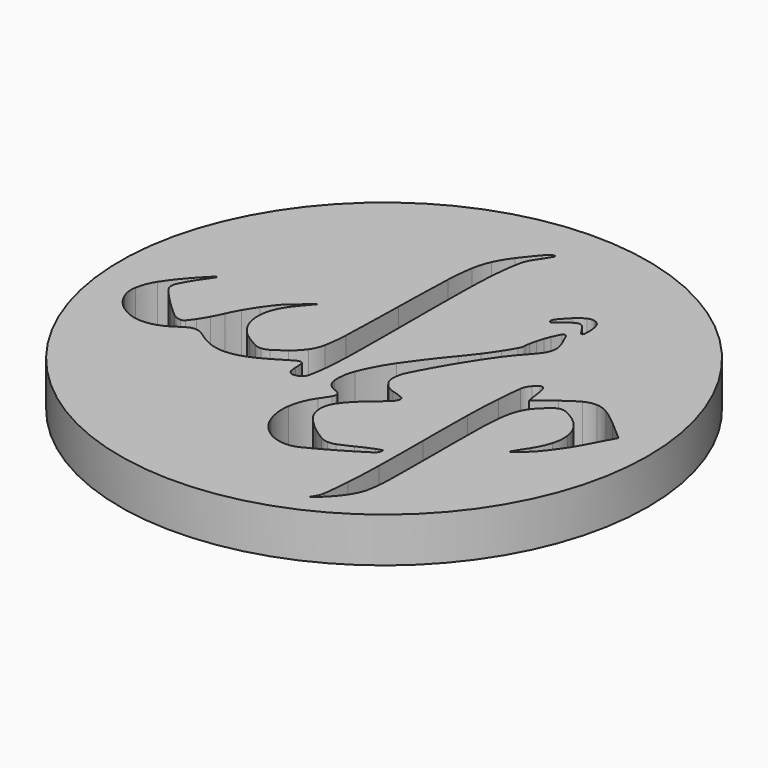
from build123d import *

# Parameters (mm, degrees)
F0_R     = 37.4493495169
F1_DEPTH = 6.35


# Not quite as in the source:
# - ends of sketch curves that miss each other by under 0.0002 mm in the source are joined


with BuildPart() as f1:
    # F0 (on Top) → F1 (new body)
    with BuildSketch(Plane.XY):
        Circle(F0_R)
        with BuildLine():
            ThreePointArc((10.8762792992, 14.7634018997), (11.0313140513, 15.1945068604), (11.2048912988, 15.61848587))
            ThreePointArc((11.2048912988, 15.61848587), (11.4768149901, 16.2225478114), (11.7640170164, 16.8194969919))
            ThreePointArc((11.7640170164, 16.8194969919), (11.8893481048, 16.9475361559), (12.0659669633, 16.9776647483))
            ThreePointArc((12.0659669633, 16.9776647483), (12.2485562258, 16.9031054882), (12.3751538129, 16.7518739087))
            ThreePointArc((12.3751538129, 16.7518739087), (12.70768613, 16.0552130167), (13.0282612117, 15.3529696483))
            ThreePointArc((13.0282612117, 15.3529696483), (13.2526035183, 14.7629142618), (13.4091322236, 14.151364044))
            ThreePointArc((13.4091322236, 14.151364044), (13.4527191197, 13.6473123792), (13.3873230886, 13.1456239785))
            ThreePointArc((13.3873230886, 13.1456239785), (13.20788262, 12.622156364), (12.9350425168, 12.1407256401))
            ThreePointArc((12.9350425168, 12.1407256401), (12.4654497003, 11.5128213922), (11.954437155, 10.9181388574))
            ThreePointArc((11.954437155, 10.9181388574), (10.5977208323, 9.3370006294), (9.3535167188, 7.6658831946))
            ThreePointArc((9.3535167188, 7.6658831946), (7.9199939418, 5.5117752747), (6.5659491385, 3.3068419184))
            ThreePointArc((6.5659491385, 3.3068419184), (5.3561218351, 1.1848137262), (4.2075785231, -0.9710002691))
            ThreePointArc((4.2075785231, -0.9710002691), (3.8216929788, -2.0075200449), (3.690609, -3.105745))
            ThreePointArc((3.690609, -3.105745), (3.7283068737, -3.4979838686), (3.8400200101, -3.8758629959))
            ThreePointArc((3.8400200101, -3.8758629959), (4.0285012326, -4.2562241711), (4.272961992, -4.6032670066))
            ThreePointArc((4.272961992, -4.6032670066), (4.574824271, -4.917630684), (4.9200760102, -5.1836129845))
            ThreePointArc((4.9200760102, -5.1836129845), (5.2913337091, -5.3865761409), (5.6906089952, -5.5265960184))
            ThreePointArc((5.6906089952, -5.5265960184), (6.4648720842, -5.7622274602), (7.2180381288, -6.0584477071))
            ThreePointArc((7.2180381288, -6.0584477071), (7.4657520558, -6.2976772359), (7.498624445, -6.6404778535))
            ThreePointArc((7.498624445, -6.6404778535), (7.3057418512, -7.0923112563), (6.9913608485, -7.4698318311))
            ThreePointArc((6.9913608485, -7.4698318311), (5.822940269, -8.5010016157), (4.6384584815, -9.5136815722))
            ThreePointArc((4.6384584815, -9.5136815722), (3.5443912184, -10.5668326908), (2.6004474224, -11.7564042914))
            ThreePointArc((2.6004474224, -11.7564042914), (2.1120521618, -12.7752539981), (1.962080368, -13.8951169912))
            ThreePointArc((1.962080368, -13.8951169912), (2.1657330329, -15.0003544038), (2.7035807171, -15.9871392184))
            ThreePointArc((2.7035807171, -15.9871392184), (3.7010773675, -17.1109770699), (4.8426470957, -18.0881308713))
            ThreePointArc((4.8426470957, -18.0881308713), (5.6504419064, -18.6581957262), (6.4856560106, -19.1872739822))
            ThreePointArc((6.4856560106, -19.1872739822), (7.0039493082, -19.4207975991), (7.5621359772, -19.5284493064))
            ThreePointArc((7.5621359772, -19.5284493064), (8.1400728978, -19.506565557), (8.6987199814, -19.3568879527))
            ThreePointArc((8.6987199814, -19.3568879527), (9.6550491416, -18.9570661492), (10.5926469221, -18.5151008439))
            ThreePointArc((10.5926469221, -18.5151008439), (11.1841988634, -18.2269156279), (11.7810690718, -17.9499131586))
            ThreePointArc((11.7810690718, -17.9499131586), (12.2773531843, -17.7352351951), (12.7805830392, -17.5373861048))
            ThreePointArc((12.7805830392, -17.5373861048), (13.1715302022, -17.3967091194), (13.5658320421, -17.2657291322))
            ThreePointArc((13.5658320421, -17.2657291322), (13.6513741496, -17.2796593868), (13.690609, -17.356939))
            ThreePointArc((13.690609, -17.356939), (13.5507780415, -17.9021018073), (13.1658118907, -18.3126578281))
            ThreePointArc((13.1658118907, -18.3126578281), (11.4102059781, -19.4044531735), (9.6328741998, -20.4605123442))
            ThreePointArc((9.6328741998, -20.4605123442), (7.8688014367, -21.4508314838), (6.0767982834, -22.3896655605))
            ThreePointArc((6.0767982834, -22.3896655605), (5.2070875666, -22.7082001651), (4.287215, -22.816345))
            ThreePointArc((4.287215, -22.816345), (2.6899630934, -22.5565730644), (1.2573490722, -21.804035904))
            ThreePointArc((1.2573490722, -21.804035904), (0.0637639813, -20.6069080986), (-0.7466320594, -19.1233250222))
            ThreePointArc((-0.7466320594, -19.1233250222), (-1.1677453841, -17.3401224067), (-1.1306904032, -15.5082449406))
            ThreePointArc((-1.1306904032, -15.5082449406), (-0.6419235107, -13.6890343723), (0.2526270965, -12.0312650676))
            ThreePointArc((0.2526270965, -12.0312650676), (0.7024614657, -11.3697564368), (1.1338345481, -10.6960637194))
            ThreePointArc((1.1338345481, -10.6960637194), (1.2685581494, -10.3917546236), (1.314644, -10.062163))
            ThreePointArc((1.314644, -10.062163), (1.2505882613, -9.810269569), (1.0739838069, -9.6195752982))
            ThreePointArc((1.0739838069, -9.6195752982), (0.6741945934, -9.38926579), (0.252626854, -9.2017703805))
            ThreePointArc((0.252626854, -9.2017703805), (-0.6381425922, -8.5264459955), (-1.0293586268, -7.4793150473))
            ThreePointArc((-1.0293586268, -7.4793150473), (-0.9713565511, -5.919909632), (-0.5670643499, -4.4127078625))
            ThreePointArc((-0.5670643499, -4.4127078625), (0.4843111612, -2.1378621147), (1.7936783431, -0.0010722388))
            ThreePointArc((1.7936783431, -0.0010722388), (3.8757468093, 2.856172185), (6.0790169795, 5.621033017))
            ThreePointArc((6.0790169795, 5.621033017), (6.8827913662, 6.6129347591), (7.6597352065, 7.625989846))
            ThreePointArc((7.6597352065, 7.625989846), (8.3503282831, 8.5851668879), (9.0081988691, 9.5670760845))
            ThreePointArc((9.0081988691, 9.5670760845), (9.526996254, 10.3975433886), (10.0205543041, 11.2432543922))
            ThreePointArc((10.0205543041, 11.2432543922), (10.199239966, 11.6673986677), (10.27697651, 12.1210329718))
            ThreePointArc((10.27697651, 12.1210329718), (10.3103188192, 12.490680364), (10.3692449003, 12.857120823))
            ThreePointArc((10.3692449003, 12.857120823), (10.4695885331, 13.3268146141), (10.585177224, 13.7929909406))
            ThreePointArc((10.585177224, 13.7929909406), (10.7229395483, 14.2805328648), (10.8762792992, 14.7634018997))
        make_face(mode=Mode.SUBTRACT)
        with BuildLine():
            ThreePointArc((16.3309902954, 3.7992979617), (16.5333642735, 4.4728969515), (16.9406093287, 5.0463446746))
            ThreePointArc((16.9406093287, 5.0463446746), (17.2598056295, 5.343826229), (17.6018882418, 5.6146786679))
            ThreePointArc((17.6018882418, 5.6146786679), (17.7996980335, 5.687411325), (18.0061756932, 5.6451534092))
            ThreePointArc((18.0061756932, 5.6451534092), (18.1901775594, 5.4936170925), (18.2964146053, 5.2802308984))
            ThreePointArc((18.2964146053, 5.2802308984), (18.4172751076, 4.757844237), (18.512282531, 4.2301429274))
            Line((18.512282531, 4.2301429274), (18.833957, 2.151252))
            Line((18.833957, 2.151252), (21.397142, 4.167454))
            ThreePointArc((21.397142, 4.167454), (22.4923393479, 4.9580300918), (23.6489884371, 5.6556192026))
            ThreePointArc((23.6489884371, 5.6556192026), (24.4741003602, 5.9692708509), (25.3534839934, 6.0458978723))
            ThreePointArc((25.3534839934, 6.0458978723), (26.2473925362, 5.8817071), (27.0687353681, 5.4925705707))
            ThreePointArc((27.0687353681, 5.4925705707), (28.2571790367, 4.6657006768), (29.3848450562, 3.757691065))
            Line((29.3848450562, 3.757691065), (32.190609, 1.331727))
            Line((32.190609, 1.331727), (30.296248, -2.217966))
            ThreePointArc((30.296248, -2.217966), (29.8748039715, -2.9711936195), (29.4237215636, -3.7070547204))
            ThreePointArc((29.4237215636, -3.7070547204), (28.9078737011, -4.4849173273), (28.3677878465, -5.2461508874))
            ThreePointArc((28.3677878465, -5.2461508874), (27.8427259014, -5.9385103963), (27.2957506754, -6.6136917283))
            ThreePointArc((27.2957506754, -6.6136917283), (26.8611052315, -7.0949015101), (26.3914461694, -7.5420031919))
            ThreePointArc((26.3914461694, -7.5420031919), (25.6864160048, -8.1620933021), (24.979266979, -8.7797659759))
            ThreePointArc((24.979266979, -8.7797659759), (24.9099925614, -8.7951216813), (24.8594533271, -8.7453169008))
            ThreePointArc((24.8594533271, -8.7453169008), (24.8509309758, -8.637712529), (24.8881566091, -8.5363933884))
            ThreePointArc((24.8881566091, -8.5363933884), (25.4995896841, -7.5796648027), (26.1129343447, -6.6241605785))
            ThreePointArc((26.1129343447, -6.6241605785), (26.7661686916, -5.4325781155), (27.2462296984, -4.1613089097))
            ThreePointArc((27.2462296984, -4.1613089097), (27.4657691357, -2.9950770933), (27.4378427219, -1.8086899068))
            ThreePointArc((27.4378427219, -1.8086899068), (27.1700390601, -0.7322913639), (26.6628924871, 0.2541946563))
            ThreePointArc((26.6628924871, 0.2541946563), (25.9198905189, 1.1553031996), (25.0139108115, 1.8923577146))
            ThreePointArc((25.0139108115, 1.8923577146), (24.3770565009, 2.28252617), (23.7150840631, 2.6283691314))
            ThreePointArc((23.7150840631, 2.6283691314), (23.2943006235, 2.7577930414), (22.8540629043, 2.7580246401))
            ThreePointArc((22.8540629043, 2.7580246401), (22.4102098559, 2.6293294742), (22.0161851262, 2.3878498451))
            ThreePointArc((22.0161851262, 2.3878498451), (21.3756572026, 1.8383388903), (20.7639108044, 1.2569571956))
            ThreePointArc((20.7639108044, 1.2569571956), (20.1177126912, 0.4779983542), (19.6265125546, -0.4069148044))
            ThreePointArc((19.6265125546, -0.4069148044), (19.2490785938, -1.4585132195), (19.0204482398, -2.552151033))
            ThreePointArc((19.0204482398, -2.552151033), (18.8311079762, -4.3239318853), (18.7496716179, -6.1039389941))
            ThreePointArc((18.7496716179, -6.1039389941), (18.7053745197, -9.9521401876), (18.690609, -13.800568))
            ThreePointArc((18.690609, -13.800568), (18.6766098173, -18.0136665407), (18.634611, -22.226579))
            ThreePointArc((18.634611, -22.226579), (18.5483521208, -23.8515074769), (18.3333395333, -25.4644559188))
            ThreePointArc((18.3333395333, -25.4644559188), (18.0420774391, -26.532147306), (17.5563022349, -27.5265421435))
            ThreePointArc((17.5563022349, -27.5265421435), (16.8067801698, -28.6115975468), (15.9406085284, -29.6060195403))
            ThreePointArc((15.9406085284, -29.6060195403), (15.4455501352, -30.1087206825), (14.9453633663, -30.606319372))
            ThreePointArc((14.9453633663, -30.606319372), (14.6624168408, -30.8702392299), (14.3656094129, -31.1184685217))
            ThreePointArc((14.3656094129, -31.1184685217), (14.3129853823, -31.1201666484), (14.2959902827, -31.0703337714))
            ThreePointArc((14.2959902827, -31.0703337714), (14.3563319607, -30.9254529061), (14.440608935, -30.7930559503))
            ThreePointArc((14.440608935, -30.7930559503), (14.8362431246, -30.1040045579), (15.0387326922, -29.3356840876))
            ThreePointArc((15.0387326922, -29.3356840876), (15.2438875337, -27.5063149861), (15.396833155, -25.6718430107))
            ThreePointArc((15.396833155, -25.6718430107), (15.5444692897, -23.0388071022), (15.6240356417, -20.4028359938))
            ThreePointArc((15.6240356417, -20.4028359938), (15.6739642523, -16.5453635979), (15.690609, -12.687604))
            ThreePointArc((15.690609, -12.687604), (15.7066642084, -8.7823894999), (15.754827005, -4.877439))
            ThreePointArc((15.754827005, -4.877439), (15.8320341926, -2.2982460629), (15.9787460161, 0.2779279989))
            ThreePointArc((15.9787460161, 0.2779279989), (16.1290481704, 2.0411957676), (16.3309902954, 3.7992979617))
        make_face(mode=Mode.SUBTRACT)
        with BuildLine():
            ThreePointArc((-5.1638240927, 25.4968420429), (-4.5115373025, 26.726620205), (-3.7290150689, 27.8779200526))
            ThreePointArc((-3.7290150689, 27.8779200526), (-2.8034988222, 29.0619061444), (-1.8501204762, 30.2235744004))
            ThreePointArc((-1.8501204762, 30.2235744004), (-1.352389791, 30.7150837207), (-0.7726823688, 31.1065636729))
            ThreePointArc((-0.7726823688, 31.1065636729), (-0.5642515513, 31.075554039), (-0.5379862128, 30.866473123))
            ThreePointArc((-0.5379862128, 30.866473123), (-1.1246347223, 29.9006129981), (-1.7526865849, 28.9611487092))
            ThreePointArc((-1.7526865849, 28.9611487092), (-2.2577368351, 28.0484196661), (-2.560209432, 27.0500908916))
            ThreePointArc((-2.560209432, 27.0500908916), (-2.8289692659, 25.394788073), (-3.0059229332, 23.7271709948))
            ThreePointArc((-3.0059229332, 23.7271709948), (-3.1695693119, 21.0857474779), (-3.2474590092, 18.4404060001))
            ThreePointArc((-3.2474590092, 18.4404060001), (-3.2939079858, 13.7543743117), (-3.309391, 9.068138))
            ThreePointArc((-3.309391, 9.068138), (-3.3226662247, 4.2545803127), (-3.3624830025, -0.558831))
            ThreePointArc((-3.3624830025, -0.558831), (-3.4324874841, -2.9906997659), (-3.5887564197, -5.4185519655))
            ThreePointArc((-3.5887564197, -5.4185519655), (-3.7490976792, -6.8280257808), (-3.9971544633, -8.2247339027))
            ThreePointArc((-3.9971544633, -8.2247339027), (-4.2819047726, -8.8047678804), (-4.809390914, -9.1779712242))
            ThreePointArc((-4.809390914, -9.1779712242), (-5.1348193627, -9.2718618438), (-5.4714800143, -9.3089924118))
            ThreePointArc((-5.4714800143, -9.3089924118), (-5.7234372186, -9.2663801944), (-5.9411163543, -9.1325363855))
            ThreePointArc((-5.9411163543, -9.1325363855), (-6.1202455253, -8.9076075266), (-6.2221577288, -8.638731943))
            ThreePointArc((-6.2221577288, -8.638731943), (-6.2875240622, -8.2214566589), (-6.309391, -7.799659))
            ThreePointArc((-6.309391, -7.799659), (-6.3304194397, -7.2188572119), (-6.3933959364, -6.6410969907))
            ThreePointArc((-6.3933959364, -6.6410969907), (-6.5071875405, -6.4344752081), (-6.7287599986, -6.353563163))
            ThreePointArc((-6.7287599986, -6.353563163), (-7.070872805, -6.4011122716), (-7.3893717582, -6.5347554156))
            ThreePointArc((-7.3893717582, -6.5347554156), (-8.4777171615, -7.1754298694), (-9.559391241, -7.8273046047))
            ThreePointArc((-9.559391241, -7.8273046047), (-10.8876430417, -8.5628076879), (-12.2727008971, -9.1847662574))
            ThreePointArc((-12.2727008971, -9.1847662574), (-13.4400666629, -9.5471793368), (-14.6499910202, -9.7208716818))
            ThreePointArc((-14.6499910202, -9.7208716818), (-15.7395021772, -9.6881211841), (-16.8039711115, -9.4535723479))
            ThreePointArc((-16.8039711115, -9.4535723479), (-17.8646396938, -9.0168818566), (-18.841863825, -8.4162577607))
            ThreePointArc((-18.841863825, -8.4162577607), (-19.3845295716, -8.0484711775), (-19.9520778071, -7.7203826369))
            ThreePointArc((-19.9520778071, -7.7203826369), (-20.3493223963, -7.5679932262), (-20.771626, -7.516172))
            ThreePointArc((-20.771626, -7.516172), (-21.1989586405, -7.5674171087), (-21.6020589665, -7.7182460648))
            ThreePointArc((-21.6020589665, -7.7182460648), (-22.1904422989, -8.0479796224), (-22.7555000671, -8.4162579042))
            ThreePointArc((-22.7555000671, -8.4162579042), (-23.7211476977, -8.9974124631), (-24.7577827037, -9.439683854))
            ThreePointArc((-24.7577827037, -9.439683854), (-25.7530511623, -9.6856291248), (-26.7764880227, -9.7458396875))
            ThreePointArc((-26.7764880227, -9.7458396875), (-27.7660616156, -9.6182800483), (-28.7136039117, -9.3057247989))
            ThreePointArc((-28.7136039117, -9.3057247989), (-29.6432492403, -8.8047594473), (-30.4806502803, -8.1613573097))
            ThreePointArc((-30.4806502803, -8.1613573097), (-31.2987000783, -7.2338340456), (-31.8892655875, -6.1472168327))
            ThreePointArc((-31.8892655875, -6.1472168327), (-32.1679131653, -5.0339528522), (-32.127810408, -3.8870469278))
            ThreePointArc((-32.127810408, -3.8870469278), (-31.7438974495, -2.5331037875), (-31.0955467738, -1.2840271482))
            ThreePointArc((-31.0955467738, -1.2840271482), (-29.9715884577, 0.2892979586), (-28.7246325537, 1.7670445915))
            ThreePointArc((-28.7246325537, 1.7670445915), (-28.066729604, 2.4785206841), (-27.4015921457, 3.1832381389))
            ThreePointArc((-27.4015921457, 3.1832381389), (-27.1086637533, 3.4602662141), (-26.788723812, 3.7056027266))
            ThreePointArc((-26.788723812, 3.7056027266), (-26.7038521522, 3.69934333), (-26.6915623806, 3.6151332236))
            ThreePointArc((-26.6915623806, 3.6151332236), (-26.9484454873, 3.2006617013), (-27.2246329596, 2.7987959708))
            ThreePointArc((-27.2246329596, 2.7987959708), (-27.6318279036, 2.2186524334), (-28.0228838324, 1.6275098924))
            ThreePointArc((-28.0228838324, 1.6275098924), (-28.3696278664, 1.0664552314), (-28.6969932193, 0.4938771205))
            ThreePointArc((-28.6969932193, 0.4938771205), (-28.953201028, 0.0097729718), (-29.1942598746, -0.482050059))
            ThreePointArc((-29.1942598746, -0.482050059), (-29.2802568297, -0.7329931815), (-29.309391, -0.996658))
            ThreePointArc((-29.309391, -0.996658), (-29.1942156301, -1.6353148627), (-28.8632007476, -2.1935057814))
            ThreePointArc((-28.8632007476, -2.1935057814), (-27.8651383232, -3.3009518322), (-26.8240056473, -4.368007642))
            ThreePointArc((-26.8240056473, -4.368007642), (-25.741392161, -5.3927215057), (-24.6187447305, -6.3734116788))
            ThreePointArc((-24.6187447305, -6.3734116788), (-24.049238313, -6.7021698615), (-23.40164, -6.816345))
            ThreePointArc((-23.40164, -6.816345), (-23.1295441915, -6.7559519585), (-22.9085491184, -6.5861149009))
            ThreePointArc((-22.9085491184, -6.5861149009), (-22.5106272783, -6.086485752), (-22.1377365637, -5.5679072977))
            ThreePointArc((-22.1377365637, -5.5679072977), (-21.7021040785, -4.8921176838), (-21.3025171091, -4.1944089412))
            ThreePointArc((-21.3025171091, -4.1944089412), (-20.8870522575, -3.3877035832), (-20.5013649128, -2.566345039))
            ThreePointArc((-20.5013649128, -2.566345039), (-20.0719321723, -1.6680560959), (-19.5977571982, -0.7925598861))
            ThreePointArc((-19.5977571982, -0.7925598861), (-19.0445725612, 0.1266080783), (-18.4547663576, 1.0227172458))
            ThreePointArc((-18.4547663576, 1.0227172458), (-17.8726251513, 1.8331854642), (-17.2575838826, 2.6189789041))
            ThreePointArc((-17.2575838826, 2.6189789041), (-16.7564297927, 3.1763915721), (-16.2045707384, 3.6836546868))
            Line((-16.2045707384, 3.6836546868), (-13.809391, 5.683655))
            Line((-13.809391, 5.683655), (-15.559391, 3.604914))
            ThreePointArc((-15.559391, 3.604914), (-16.3542818779, 2.4712676939), (-16.9378245283, 1.2156868295))
            ThreePointArc((-16.9378245283, 1.2156868295), (-17.241673479, -0.0374188601), (-17.2674484508, -1.3265790402))
            ThreePointArc((-17.2674484508, -1.3265790402), (-17.0164722734, -2.5351561469), (-16.4947934701, -3.6538602896))
            ThreePointArc((-16.4947934701, -3.6538602896), (-15.7221139093, -4.6457613104), (-14.7521508208, -5.4458067266))
            ThreePointArc((-14.7521508208, -5.4458067266), (-13.9637761936, -5.9343690501), (-13.1517401861, -6.3825043584))
            ThreePointArc((-13.1517401861, -6.3825043584), (-12.6775691786, -6.5520681186), (-12.1753060291, -6.5884225417))
            ThreePointArc((-12.1753060291, -6.5884225417), (-11.6626585181, -6.4909796815), (-11.1898354036, -6.2702063581))
            ThreePointArc((-11.1898354036, -6.2702063581), (-10.3344863457, -5.7083129064), (-9.5021506616, -5.1128604537))
            ThreePointArc((-9.5021506616, -5.1128604537), (-8.6443699796, -4.3600688618), (-7.9164820374, -3.4810569737))
            ThreePointArc((-7.9164820374, -3.4810569737), (-7.4162331381, -2.5771997991), (-7.1187463679, -1.587902931))
            ThreePointArc((-7.1187463679, -1.587902931), (-6.878296597, 0.0371012679), (-6.7635773377, 1.6757880106))
            ThreePointArc((-6.7635773377, 1.6757880106), (-6.6340649172, 6.204526973), (-6.5299067741, 10.7339199954))
            ThreePointArc((-6.5299067741, 10.7339199954), (-6.4282503718, 14.9882558314), (-6.2951489485, 19.2417239982))
            ThreePointArc((-6.2951489485, 19.2417239982), (-6.1683186308, 21.1398447912), (-5.9213269074, 23.0260959849))
            ThreePointArc((-5.9213269074, 23.0260959849), (-5.6264288282, 24.2871774873), (-5.1638240927, 25.4968420429))
        make_face(mode=Mode.SUBTRACT)
        with BuildLine():
            ThreePointArc((9.0053870761, 19.2579189344), (9.6256520715, 19.9514179813), (10.2712290627, 20.6214179373))
            ThreePointArc((10.2712290627, 20.6214179373), (10.8725535369, 21.1330477233), (11.5480517805, 21.5417754389))
            ThreePointArc((11.5480517805, 21.5417754389), (12.0984831662, 21.6882140221), (12.6618858948, 21.6045707127))
            ThreePointArc((12.6618858948, 21.6045707127), (13.1252327379, 21.3087582153), (13.4211337422, 20.8454679055))
            ThreePointArc((13.4211337422, 20.8454679055), (13.6146438867, 20.1215320353), (13.6752962492, 19.3746379977))
            ThreePointArc((13.6752962492, 19.3746379977), (13.665126071, 18.9182737222), (13.6428905433, 18.4623380283))
            ThreePointArc((13.6428905433, 18.4623380283), (13.5969199665, 18.3444292445), (13.4910222598, 18.27513606))
            ThreePointArc((13.4910222598, 18.27513606), (13.3638778055, 18.2797675976), (13.2624748994, 18.3566089287))
            ThreePointArc((13.2624748994, 18.3566089287), (13.0020226741, 18.7346510384), (12.7515123742, 19.1193532368))
            ThreePointArc((12.7515123742, 19.1193532368), (12.4975637807, 19.4791169551), (12.2086430827, 19.8114490795))
            ThreePointArc((12.2086430827, 19.8114490795), (11.9840546331, 19.9705428383), (11.7166909695, 20.0358684054))
            ThreePointArc((11.7166909695, 20.0358684054), (11.4159073599, 20.0046215603), (11.1389454023, 19.8832163694))
            ThreePointArc((11.1389454023, 19.8832163694), (10.6929549737, 19.5786718445), (10.2668240802, 19.2469079033))
            ThreePointArc((10.2668240802, 19.2469079033), (9.6728326859, 18.7829155122), (9.0524392738, 18.3548655769))
            ThreePointArc((9.0524392738, 18.3548655769), (8.8410465989, 18.3469815276), (8.73339706, 18.5290819998))
            ThreePointArc((8.73339706, 18.5290819998), (8.8042124766, 18.9178244505), (9.0053870761, 19.2579189344))
        make_face(mode=Mode.SUBTRACT)
    extrude(amount=F1_DEPTH)


solid = f1.part
